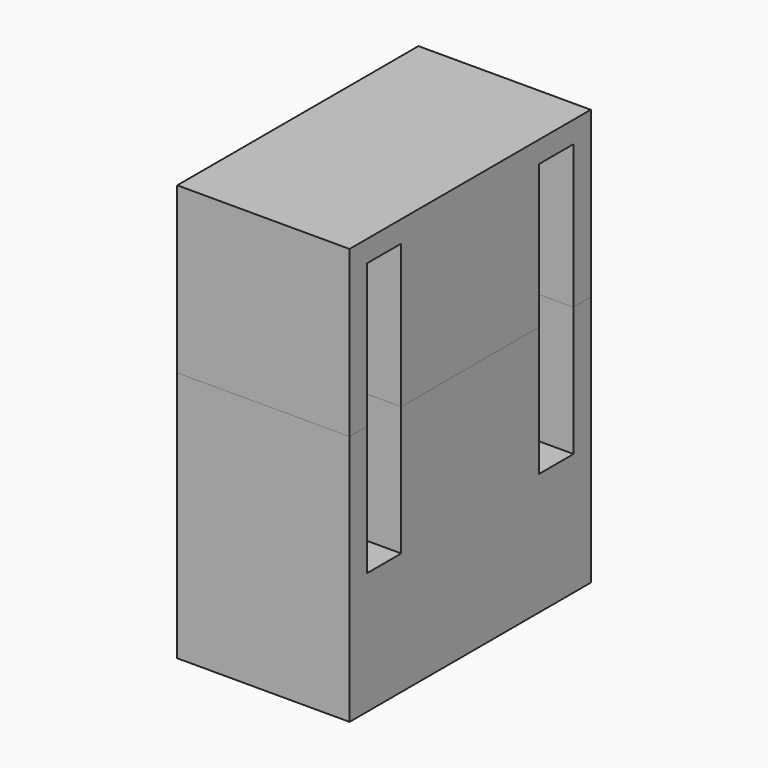
from build123d import *

# Parameters (mm, degrees)
F1_DEPTH = 10
F0_W     = 6.5
F0_H     = 12
F2_W     = 10.2
F2_H     = 18
F3_DEPTH = 1.5
F4_DEPTH = 16
F6_DEPTH = 1.5
F5_W     = 6.5
F5_H     = 3
F7_DEPTH = 1.5
F8_DEPTH = 7


# Not quite as in the source:
# - a feature names something its author has since deleted; it is built from what else it names


with BuildPart() as f1:
    # F0 (on Top) → F1 (new body)
    with BuildSketch(Plane.XY):
        Polygon((-5.6070076972, 9.0611978821), (-17.6070076972, 9.0611978821), (-17.6070076972, -11.9388021179), (-5.6070076972, -11.9388021179), (-5.6070076972, -10.4388021179), (-15.8070076972, -10.4388021179), (-15.8070076972, 7.5611978821), (-5.6070076972, 7.5611978821), align=None)
    extrude(amount=F1_DEPTH)



with BuildPart() as f1b:
    # F0 (on Top) → F1, piece 2 (new body)
    with BuildSketch(Plane.XY):
        with Locations((-8.8570076972, -1.4388021179)):
            Rectangle(F0_W, F0_H)
    extrude(amount=F1_DEPTH)


with BuildPart() as f1_1:
    add(f1.part)

    add(f1b.part)  # F3 merges F1b
    # F2 (on face) → F3 (join)
    with BuildSketch(Plane.XY.offset(10)):
        Polygon((-5.6070076972, 9.0611978821), (-17.6070076972, 9.0611978821), (-17.6070076972, -11.9388021179), (-5.6070076972, -11.9388021179), (-5.6070076972, -10.4388021179), (-15.8070076972, -10.4388021179), (-15.8070076972, 7.5611978821), (-5.6070076972, 7.5611978821), align=None)
        with Locations((-10.7070076972, -1.4388021179)):
            Rectangle(F2_W, F2_H)
    extrude(amount=F3_DEPTH)


with BuildPart() as f4:
    # F0 (on Top) → F4 (new body)
    with BuildSketch(Plane.XY):
        Polygon((-5.6070076972, 9.0611978821), (-17.6070076972, 9.0611978821), (-17.6070076972, -11.9388021179), (-5.6070076972, -11.9388021179), (-5.6070076972, -10.4388021179), (-15.8070076972, -10.4388021179), (-15.8070076972, 7.5611978821), (-5.6070076972, 7.5611978821), align=None)
    extrude(amount=-F4_DEPTH)



with BuildPart() as f4b:
    # F0 (on Top) → F4, piece 2 (new body)
    with BuildSketch(Plane.XY):
        with Locations((-8.8570076972, -1.4388021179)):
            Rectangle(F0_W, F0_H)
    extrude(amount=-F4_DEPTH)


with BuildPart() as f4_1:
    add(f4.part)

    add(f4b.part)  # F6 merges F4b
    # F5 (on face) → F6 (join)
    with BuildSketch(Plane(origin=(0, 0, -16), x_dir=(1, 0, 0), z_dir=(0, 0, -1))):
        Polygon((-5.6070076972, 11.9388021179), (-17.6070076972, 11.9388021179), (-17.6070076972, -9.0611978821), (-5.6070076972, -9.0611978821), (-5.6070076972, -7.5611978821), (-12.1070076972, -7.5611978821), (-15.8070076972, -7.5611978821), (-15.8070076972, 10.4388021179), (-12.1070076972, 10.4388021179), (-5.6070076972, 10.4388021179), align=None)
        Polygon((-5.6070076972, -4.5611978821), (-5.6070076972, 7.4388021179), (-12.1070076972, 7.4388021179), (-12.1070076972, 10.4388021179), (-15.8070076972, 10.4388021179), (-15.8070076972, -7.5611978821), (-12.1070076972, -7.5611978821), (-12.1070076972, -4.5611978821), align=None)
    extrude(amount=F6_DEPTH)

    # F5 (on face) → F7 (join)
    with BuildSketch(Plane(origin=(0, 0, -16), x_dir=(1, 0, 0), z_dir=(0, 0, -1))):
        with Locations((-8.8570076972, -6.0611978821)):
            Rectangle(F5_W, F5_H)
        with Locations((-8.8570076972, 8.9388021179)):
            Rectangle(F5_W, F5_H)
    extrude(amount=F7_DEPTH)

    # F5 (on face) → F8 (join)
    with BuildSketch(Plane(origin=(0, 0, -16), x_dir=(1, 0, 0), z_dir=(0, 0, -1))):
        with Locations((-8.8570076972, -6.0611978821)):
            Rectangle(F5_W, F5_H)
        with Locations((-8.8570076972, 8.9388021179)):
            Rectangle(F5_W, F5_H)
    extrude(amount=-F8_DEPTH)


solid = Compound([f1_1.part, f4_1.part])
